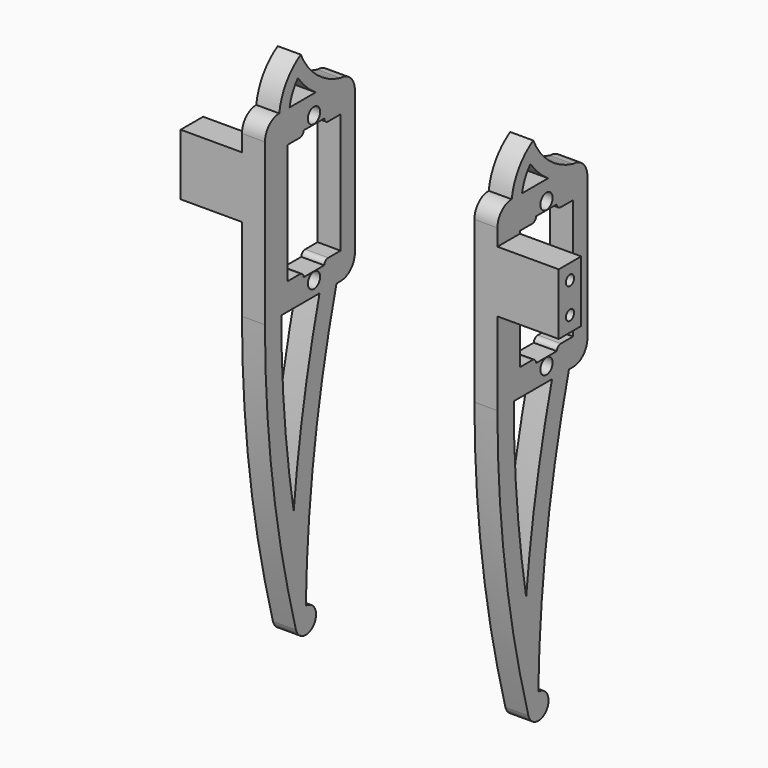
from build123d import *

# Parameters (mm, degrees)
F0_W           = 22
F0_H           = 35
F1_DEPTH       = 4.5
F3_DEPTH       = 4.5
F4_R           = 3.5
F6_DEPTH       = 4.5
F7_W           = 5.5
F7_H           = 12
F8_DEPTH       = 12
F9_W           = 13
F9_H           = 23.5
F10_DEPTH      = 25
F11_R          = 1.5
F12_DEPTH      = 25
F13_R          = 1
F14_DEPTH      = 5
F17_W          = 5
F17_H          = 0.9
F18_DEPTH      = 60
F19_T1_DEPTH   = 9.4749371855
F19_2_T1_DEPTH = 9.4749371855


# Not quite as in the source:
# - a fillet or chamfer that OpenCascade refuses, or shapes differently, is made with other operations: its cross-section is extruded or revolved along the edge and cut away or added


with BuildPart() as f1:
    # F0 (on Right) → F1 (new body)
    with BuildSketch(Plane.YZ):
        Rectangle(F0_W, F0_H)
    extrude(amount=F1_DEPTH)

    # F2 (on Right) → F3 (join, through all)
    with BuildSketch(Plane.YZ):
        with BuildLine():
            ThreePointArc((-3.4087221095, -73.1693711968), (-2.9904054853, -70.9872918312), (-1, -70))
            ThreePointArc((-1, -70), (1.1380813831, -43.5197259119), (6.5, -17.5))
            Line((6.5, -17.5), (2.3585708498, -17.5))
            ThreePointArc((2.3585708498, -17.5), (-1.5137994024, -34.8722383779), (-3.9738680642, -52.5))
            ThreePointArc((-3.9738680642, -52.5), (-6.2420584126, -35.065288743), (-7, -17.5))
            Line((-7, -17.5), (-11, -17.5))
            ThreePointArc((-11, -17.5), (-9.0934391059, -45.5922871508), (-3.4087221095, -73.1693711968))
        make_face()
        with BuildLine():
            ThreePointArc((-3.4087221095, -73.1693711968), (-0.6622169882, -74.9770754201), (1.5, -72.5))
            ThreePointArc((1.5, -72.5), (0.767766953, -70.732233047), (-1, -70))
            ThreePointArc((-1, -70), (-2.9904054853, -70.9872918312), (-3.4087221095, -73.1693711968))
        make_face()
    extrude(amount=F3_DEPTH)

    # F4
    f4_edges = [f1.edges().sort_by_distance(p)[0] for p in [
        (2.25, -11, 17.5),
        (2.25, 11, 17.5),
        (2.25, 11, -17.5),
    ]]
    fillet(f4_edges, radius=F4_R)

    # F5 (on Right) → F6 (join, through all)
    with BuildSketch(Plane.YZ):
        with BuildLine():
            Line((1.4, 17.5), (7.5, 17.5))
            ThreePointArc((7.5, 17.5), (1.7091044965, 20.3837523551), (-2.25, 25.5))
            ThreePointArc((-2.25, 25.5), (-5.7904576912, 22.1007691099), (-7.5, 17.5))
            Line((-7.5, 17.5), (-4.9720180544, 17.5))
            ThreePointArc((-4.9720180544, 17.5), (-4.2510603876, 19.7558550861), (-2.9356909086, 21.7252370349))
            ThreePointArc((-2.9356909086, 21.7252370349), (-0.9575351482, 19.4179700576), (1.4, 17.5))
        make_face()
    extrude(amount=F6_DEPTH)

    # F7 (on face) → F8 (join)
    with BuildSketch(Plane(origin=(0, 0, 0), x_dir=(0, -1, 0), z_dir=(-1, 0, 0))):
        with Locations((8.25, 4.75)):
            Rectangle(F7_W, F7_H)
    extrude(amount=F8_DEPTH)

    # F9 (on face) → F10 (cut)
    with BuildSketch(Plane(origin=(0, 0, 0), x_dir=(0, -1, 0), z_dir=(-1, 0, 0))):
        with Locations((-1, -0.5)):
            Rectangle(F9_W, F9_H)
    extrude(amount=-F10_DEPTH, mode=Mode.SUBTRACT)

    # F11 (on face) → F12 (cut)
    with BuildSketch(Plane(origin=(0, 0, 0), x_dir=(0, -1, 0), z_dir=(-1, 0, 0))):
        with Locations((-1, 13.7)):
            Circle(F11_R)
        with Locations((-1, -14.7)):
            Circle(F11_R)
    extrude(amount=-F12_DEPTH, mode=Mode.SUBTRACT)

    # F13 (on face) → F14 (cut)
    with BuildSketch(Plane(origin=(-12, 0, 0), x_dir=(0, -1, 0), z_dir=(-1, 0, 0))):
        with Locations((8.25, 7.75)):
            Circle(F13_R)
        with Locations((8.25, 1.75)):
            Circle(F13_R)
    extrude(amount=-F14_DEPTH, mode=Mode.SUBTRACT)


with BuildPart() as f16_1:
    # F16: instance of F1
    add(f1.part.mirror(Plane.YZ.offset(25)))


with BuildPart() as f18_tool:
    # F17 (on face) → F18 (new body)
    with BuildSketch(Plane.YZ.offset(50)):
        with Locations((1, 11.7)):
            Rectangle(F17_W, F17_H)
        with Locations((1, -12.7)):
            Rectangle(F17_W, F17_H)
    extrude(amount=-F18_DEPTH)


with BuildPart() as f1_1:
    add(f1.part)

    # F18: cut by f18_tool
    add(f18_tool.part, mode=Mode.SUBTRACT)

    # F19: fillet of radius 1 on 4 edges, made by hand

    # F19_s2 → F19_t1 (cut)
    with BuildSketch(Plane.YZ.offset(-2.4874685928)):
        with BuildLine():
            ThreePointArc((-1.5, 12.15), (-1.8241670439, 11.5083801513), (-2.4949874371, 11.25))
            Line((-2.4949874371, 11.25), (-1.5, 11.25))
            Line((-1.5, 11.25), (-1.5, 12.15))
        make_face()
        with BuildLine():
            ThreePointArc((4.4949874371, 11.25), (3.8241670439, 11.5083801513), (3.5, 12.15))
            Line((3.5, 12.15), (3.5, 11.25))
            Line((3.5, 11.25), (4.4949874371, 11.25))
        make_face()
        with BuildLine():
            ThreePointArc((3.5, -13.15), (3.8241670439, -12.5083801513), (4.4949874371, -12.25))
            Line((4.4949874371, -12.25), (3.5, -12.25))
            Line((3.5, -12.25), (3.5, -13.15))
        make_face()
        with BuildLine():
            ThreePointArc((-2.4949874371, -12.25), (-1.8241670439, -12.5083801513), (-1.5, -13.15))
            Line((-1.5, -13.15), (-1.5, -12.25))
            Line((-1.5, -12.25), (-2.4949874371, -12.25))
        make_face()
    extrude(amount=F19_T1_DEPTH, mode=Mode.SUBTRACT)


with BuildPart() as f16_1_1:
    add(f16_1.part)

    # F18: cut by f18_tool
    add(f18_tool.part, mode=Mode.SUBTRACT)

    # F19#2: fillet of radius 1 on 4 edges, made by hand

    # F19_2_s2 → F19_2_t1 (cut)
    with BuildSketch(Plane.YZ.offset(43.0125314072)):
        with BuildLine():
            ThreePointArc((-1.5, 12.15), (-1.8241670439, 11.5083801513), (-2.4949874371, 11.25))
            Line((-2.4949874371, 11.25), (-1.5, 11.25))
            Line((-1.5, 11.25), (-1.5, 12.15))
        make_face()
        with BuildLine():
            ThreePointArc((4.4949874371, 11.25), (3.8241670439, 11.5083801513), (3.5, 12.15))
            Line((3.5, 12.15), (3.5, 11.25))
            Line((3.5, 11.25), (4.4949874371, 11.25))
        make_face()
        with BuildLine():
            ThreePointArc((-2.4949874371, -12.25), (-1.8241670439, -12.5083801513), (-1.5, -13.15))
            Line((-1.5, -13.15), (-1.5, -12.25))
            Line((-1.5, -12.25), (-2.4949874371, -12.25))
        make_face()
        with BuildLine():
            ThreePointArc((3.5, -13.15), (3.8241670439, -12.5083801513), (4.4949874371, -12.25))
            Line((4.4949874371, -12.25), (3.5, -12.25))
            Line((3.5, -12.25), (3.5, -13.15))
        make_face()
    extrude(amount=F19_2_T1_DEPTH, mode=Mode.SUBTRACT)


solid = Compound([f1_1.part, f16_1_1.part])
